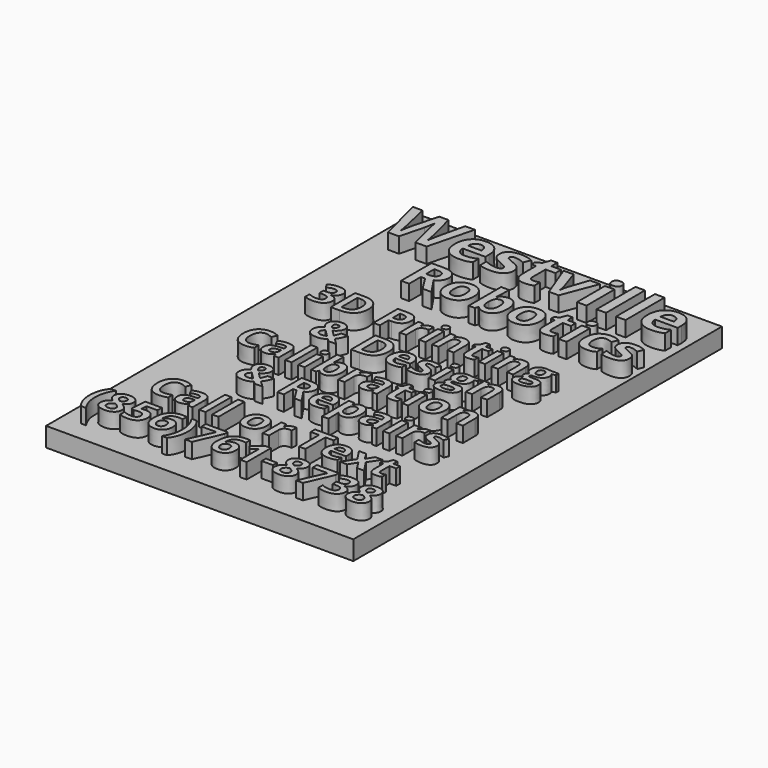
from build123d import *

# Parameters (mm, degrees)
F0_W           = 50.8
F0_H           = 76.2
F1_DEPTH       = 3.175
F2_TEXT_SIZE   = 10.5833333333
F2_TEXT_SIZE_2 = 8.8194444444
F2_TEXT_SIZE_3 = 7.0555555556
F3_DEPTH       = 2.54


# Not quite as in the source:
# - Text() gives the source's letters only with a copy of the font that has no kerning and outlines rounded to 1/6400 em; it was checked with that copy


with BuildPart() as f1:
    # F0 (on Top) → F1 (new body)
    with BuildSketch(Plane.XY):
        Rectangle(F0_W, F0_H)
    extrude(amount=F1_DEPTH)

    # F2 (on face) → F3 (join)
    with BuildSketch(Plane.XY.offset(3.175)):
        with Locations((-23.622, 27.94)):
            Text('Westville', F2_TEXT_SIZE, font='Open Sans', font_style=FontStyle.BOLD, text_align=(TextAlign.LEFT, TextAlign.BOTTOM))
        with Locations((-12.7, 18.415)):
            Text('Robotics', F2_TEXT_SIZE_2, font='Open Sans', font_style=FontStyle.BOLD, text_align=(TextAlign.LEFT, TextAlign.BOTTOM))
        with Locations((-19.05, 6.985)):
            Text('3D Printing', F2_TEXT_SIZE_3, font='Open Sans', font_style=FontStyle.BOLD, text_align=(TextAlign.LEFT, TextAlign.BOTTOM))
        with Locations((-12.7, -0.635)):
            Text('& Design', F2_TEXT_SIZE_3, font='Open Sans', font_style=FontStyle.BOLD, text_align=(TextAlign.LEFT, TextAlign.BOTTOM))
        with Locations((-19.05, -8.255)):
            Text('Calibration', F2_TEXT_SIZE_3, font='Open Sans', font_style=FontStyle.BOLD, text_align=(TextAlign.LEFT, TextAlign.BOTTOM))
        with Locations((-12.7, -15.875)):
            Text('& Repairs', F2_TEXT_SIZE_3, font='Open Sans', font_style=FontStyle.BOLD, text_align=(TextAlign.LEFT, TextAlign.BOTTOM))
        with Locations((-23.622, -33.655)):
            Text('(856)761-8738', F2_TEXT_SIZE_3, font='Open Sans', font_style=FontStyle.BOLD, text_align=(TextAlign.LEFT, TextAlign.BOTTOM))
        with Locations((-19.05, -26.035)):
            Text('Call or Text', F2_TEXT_SIZE_3, font='Open Sans', font_style=FontStyle.BOLD, text_align=(TextAlign.LEFT, TextAlign.BOTTOM))
    extrude(amount=F3_DEPTH)


solid = f1.part
